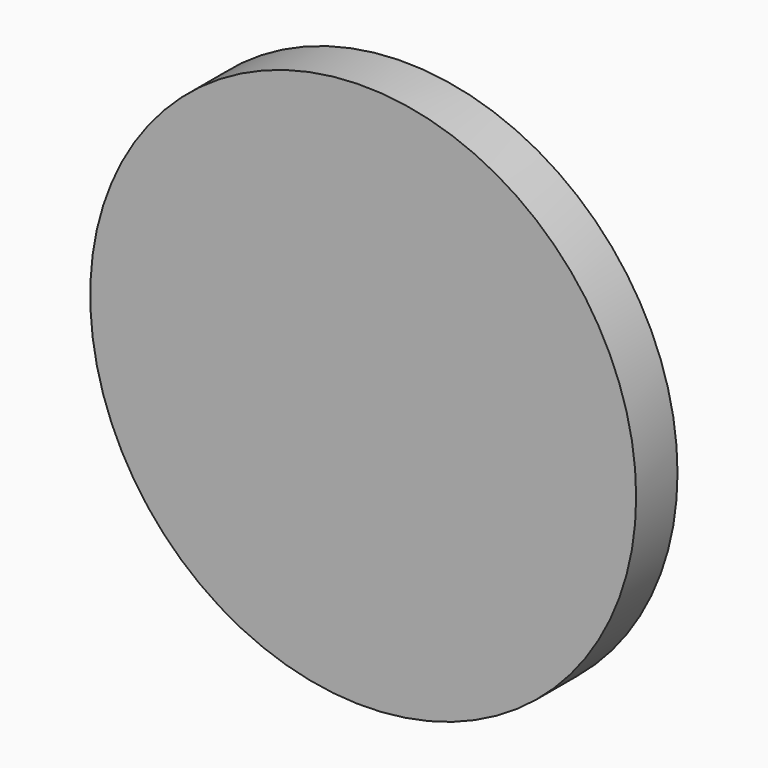
from build123d import *

# Parameters (mm, degrees)
F0_R     = 134.1311992542
F1_DEPTH = 25.4


# Not quite as in the source:
# - the program builds the solid bodies; features that only make, move or delete a surface that nothing else refers to are left out


with BuildPart() as f1:
    # F0 (on Front) → F1 (new body)
    with BuildSketch(Plane.XZ):
        Circle(F0_R)
    extrude(amount=F1_DEPTH)


solid = f1.part
